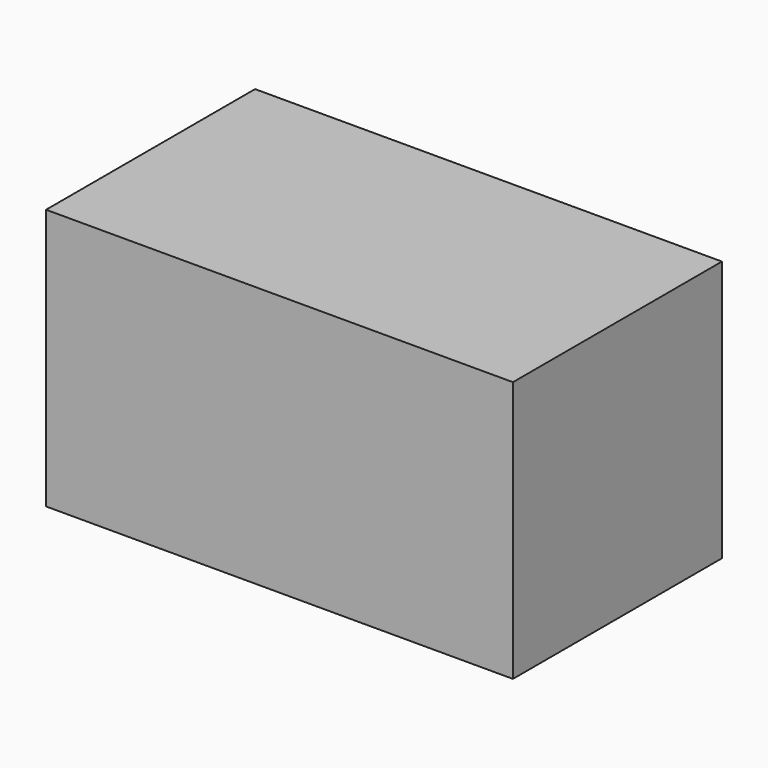
from build123d import *

# Parameters (mm, degrees)
F1_E0_TOP_W = 45.3921966255
F1_E0_TOP_H = 25.4
F2_DEPTH    = 25.4


with BuildPart() as f2:
    # F1_E0_top (on explicit) → F2 (new body)
    with BuildSketch(Plane(origin=(0, 35.1130329072, 0), x_dir=(-1, 0, 0), z_dir=(0, 1, 0))):
        with Locations((22.6960983127, 12.7)):
            Rectangle(F1_E0_TOP_W, F1_E0_TOP_H)
    extrude(amount=F2_DEPTH)


solid = f2.part
